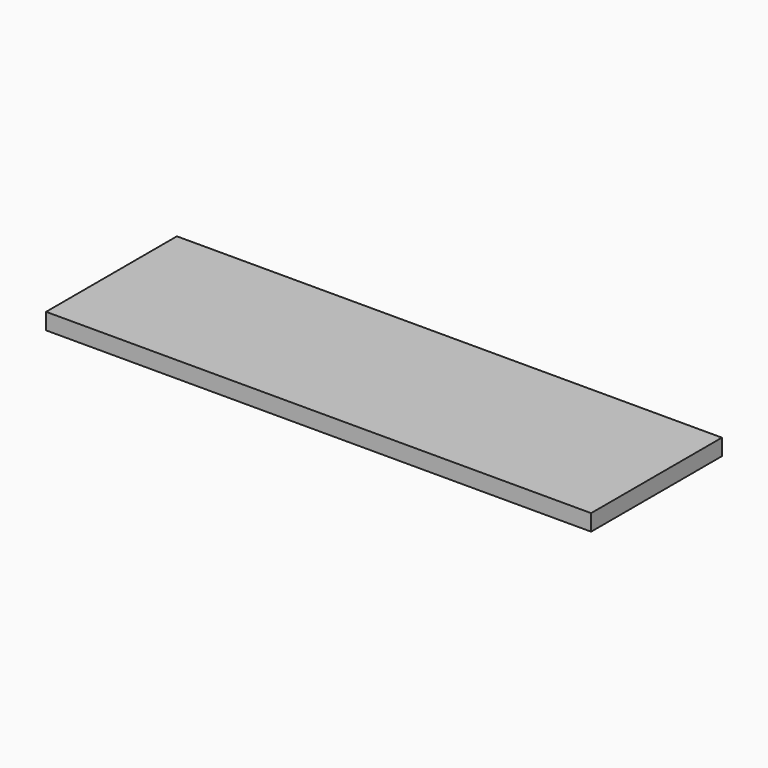
from build123d import *

# Parameters (mm, degrees)
F0_W         = 100
F0_H         = 30
F0_TEXT_SIZE = 22.2058377066
F1_DEPTH     = 2
F2_DEPTH     = 1
F3_W         = 100
F3_H         = 30
F4_DEPTH     = 1


# Not quite as in the source:
# - Text() gives the source's letters only with a copy of the font that has no kerning and outlines rounded to 1/6400 em; it was checked with that copy


with BuildPart() as f1:
    # F0 (on Top) → F1 (new body)
    with BuildSketch(Plane.XY):
        with Locations((-2.6432406157, 9.3667145638)):
            Rectangle(F0_W, F0_H)
        with BuildLine():
            add(Edge.make_bspline(
                [(-36.3527431529, 17.219600889), (-30.4126815664, 17.219600889), (-30.4126815664, 12.6014805785)],
                knots=[0, 0, 0, 1, 1, 1], degree=2))
            add(Edge.make_bspline(
                [(-30.4126815664, 12.6014805785), (-30.4126815664, 10.1935350521), (-32.0555665905, 8.8976162422)],
                knots=[0, 0, 0, 1, 1, 1], degree=2))
            add(Edge.make_bspline(
                [(-32.0555665905, 8.8976162422), (-33.6984516146, 7.6016974323), (-36.7552239613, 7.6016974323)],
                knots=[0, 0, 0, 1, 1, 1], degree=2))
            Line((-36.7552239613, 7.6016974323), (-38.6219021936, 7.6016974323))
            Line((-38.6219021936, 7.6016974323), (-38.6219021936, 1.3667145638))
            Line((-38.6219021936, 1.3667145638), (-40.4642927908, 1.3667145638))
            Line((-40.4642927908, 1.3667145638), (-40.4642927908, 17.219600889))
            Line((-40.4642927908, 17.219600889), (-36.3527431529, 17.219600889))
        make_face(mode=Mode.SUBTRACT)
        with BuildLine():
            add(Edge.make_bspline(
                [(-23.9938066044, 12.8391524352), (-23.0604674883, 13.4688961139), (-21.9432362786, 13.4688961139)],
                knots=[0, 0, 0, 1, 1, 1], degree=2))
            add(Edge.make_bspline(
                [(-21.9432362786, 13.4688961139), (-21.1521533104, 13.4688961139), (-20.5241444627, 13.3370489525)],
                knots=[0, 0, 0, 1, 1, 1], degree=2))
            Line((-20.5241444627, 13.3370489525), (-20.7739601369, 11.6681414623))
            add(Edge.make_bspline(
                [(-20.7739601369, 11.6681414623), (-21.5095285109, 11.831215583), (-22.07508344, 11.831215583)],
                knots=[0, 0, 0, 1, 1, 1], degree=2))
            add(Edge.make_bspline(
                [(-22.07508344, 11.831215583), (-23.518462891, 11.831215583), (-24.5420132227, 10.6602046102)],
                knots=[0, 0, 0, 1, 1, 1], degree=2))
            add(Edge.make_bspline(
                [(-24.5420132227, 10.6602046102), (-25.5655635545, 9.4891936374), (-25.5655635545, 7.7439535801)],
                knots=[0, 0, 0, 1, 1, 1], degree=2))
            Line((-25.5655635545, 7.7439535801), (-25.5655635545, 1.3667145638))
            Line((-25.5655635545, 1.3667145638), (-27.366318206, 1.3667145638))
            Line((-27.366318206, 1.3667145638), (-27.366318206, 13.2503073989))
            Line((-27.366318206, 13.2503073989), (-25.8813028094, 13.2503073989))
            Line((-25.8813028094, 13.2503073989), (-25.6731230809, 11.0505416011))
            Line((-25.6731230809, 11.0505416011), (-25.5863815274, 11.0505416011))
            add(Edge.make_bspline(
                [(-25.5863815274, 11.0505416011), (-24.9271457205, 12.2094087564), (-23.9938066044, 12.8391524352)],
                knots=[0, 0, 0, 1, 1, 1], degree=2))
        make_face(mode=Mode.SUBTRACT)
        with BuildLine():
            add(Edge.make_bspline(
                [(-9.5131716562, 11.8086627791), (-8.0437697392, 10.1484294443), (-8.0437697392, 7.3206547989)],
                knots=[0, 0, 0, 1, 1, 1], degree=2))
            add(Edge.make_bspline(
                [(-8.0437697392, 7.3206547989), (-8.0437697392, 4.4130779242), (-9.5062323319, 2.7806018865)],
                knots=[0, 0, 0, 1, 1, 1], degree=2))
            add(Edge.make_bspline(
                [(-9.5062323319, 2.7806018865), (-10.9686949246, 1.1481258489), (-13.550123558, 1.1481258489)],
                knots=[0, 0, 0, 1, 1, 1], degree=2))
            add(Edge.make_bspline(
                [(-13.550123558, 1.1481258489), (-15.1461681432, 1.1481258489), (-16.3813678656, 1.8975728715)],
                knots=[0, 0, 0, 1, 1, 1], degree=2))
            add(Edge.make_bspline(
                [(-16.3813678656, 1.8975728715), (-17.616567588, 2.6470198941), (-18.2896820435, 4.0452937371)],
                knots=[0, 0, 0, 1, 1, 1], degree=2))
            add(Edge.make_bspline(
                [(-18.2896820435, 4.0452937371), (-18.962796499, 5.4435675802), (-18.962796499, 7.3206547989)],
                knots=[0, 0, 0, 1, 1, 1], degree=2))
            add(Edge.make_bspline(
                [(-18.962796499, 7.3206547989), (-18.962796499, 10.2247620114), (-17.5090080616, 11.8468290626)],
                knots=[0, 0, 0, 1, 1, 1], degree=2))
            add(Edge.make_bspline(
                [(-17.5090080616, 11.8468290626), (-16.0552196243, 13.4688961139), (-13.4737909909, 13.4688961139)],
                knots=[0, 0, 0, 1, 1, 1], degree=2))
            add(Edge.make_bspline(
                [(-13.4737909909, 13.4688961139), (-10.9825735732, 13.4688961139), (-9.5131716562, 11.8086627791)],
                knots=[0, 0, 0, 1, 1, 1], degree=2))
        make_face(mode=Mode.SUBTRACT)
        with BuildLine():
            add(Edge.make_bspline(
                [(-2.4472047047, 3.2108399921), (-1.9371643699, 2.6366109076), (-1.0489308616, 2.6366109076)],
                knots=[0, 0, 0, 1, 1, 1], degree=2))
            add(Edge.make_bspline(
                [(-1.0489308616, 2.6366109076), (-0.5701174861, 2.6366109076), (-0.126000732, 2.7060041505)],
                knots=[0, 0, 0, 1, 1, 1], degree=2))
            add(Edge.make_bspline(
                [(-0.126000732, 2.7060041505), (0.3181160222, 2.7753973933), (0.5783406828, 2.8517299604)],
                knots=[0, 0, 0, 1, 1, 1], degree=2))
            Line((0.5783406828, 2.8517299604), (0.5783406828, 1.4742740902))
            add(Edge.make_bspline(
                [(0.5783406828, 1.4742740902), (0.2868890629, 1.3354876045), (-0.2821355283, 1.2418067267)],
                knots=[0, 0, 0, 1, 1, 1], degree=2))
            add(Edge.make_bspline(
                [(-0.2821355283, 1.2418067267), (-0.8511601196, 1.1481258489), (-1.3091555223, 1.1481258489)],
                knots=[0, 0, 0, 1, 1, 1], degree=2))
            add(Edge.make_bspline(
                [(-1.3091555223, 1.1481258489), (-4.7545300289, 1.1481258489), (-4.7545300289, 4.7808621112)],
                knots=[0, 0, 0, 1, 1, 1], degree=2))
            Line((-4.7545300289, 4.7808621112), (-4.7545300289, 11.8520335559))
            Line((-4.7545300289, 11.8520335559), (-6.4581341405, 11.8520335559))
            Line((-6.4581341405, 11.8520335559), (-6.4581341405, 12.7194490913))
            Line((-6.4581341405, 12.7194490913), (-4.7545300289, 13.4688961139))
            Line((-4.7545300289, 13.4688961139), (-3.998143682, 16.0052191394))
            Line((-3.998143682, 16.0052191394), (-2.9572450395, 16.0052191394))
            Line((-2.9572450395, 16.0052191394), (-2.9572450395, 13.2503073989))
            Line((-2.9572450395, 13.2503073989), (0.4915991293, 13.2503073989))
            Line((0.4915991293, 13.2503073989), (0.4915991293, 11.8520335559))
            Line((0.4915991293, 11.8520335559), (-2.9572450395, 11.8520335559))
            Line((-2.9572450395, 11.8520335559), (-2.9572450395, 4.8571946783))
            add(Edge.make_bspline(
                [(-2.9572450395, 4.8571946783), (-2.9572450395, 3.7850690765), (-2.4472047047, 3.2108399921)],
                knots=[0, 0, 0, 1, 1, 1], degree=2))
        make_face(mode=Mode.SUBTRACT)
        with BuildLine():
            add(Edge.make_bspline(
                [(10.0262306945, 1.3285482802), (9.1761634698, 1.1481258489), (7.9721907066, 1.1481258489)],
                knots=[0, 0, 0, 1, 1, 1], degree=2))
            add(Edge.make_bspline(
                [(7.9721907066, 1.1481258489), (5.3387171411, 1.1481258489), (3.8138006299, 2.7545794205)],
                knots=[0, 0, 0, 1, 1, 1], degree=2))
            add(Edge.make_bspline(
                [(3.8138006299, 2.7545794205), (2.2888841186, 4.361032992), (2.2888841186, 7.2096256103)],
                knots=[0, 0, 0, 1, 1, 1], degree=2))
            add(Edge.make_bspline(
                [(2.2888841186, 7.2096256103), (2.2888841186, 10.0859755258), (3.7045062724, 11.7774358198)],
                knots=[0, 0, 0, 1, 1, 1], degree=2))
            add(Edge.make_bspline(
                [(3.7045062724, 11.7774358198), (5.1201284262, 13.4688961139), (7.5072559797, 13.4688961139)],
                knots=[0, 0, 0, 1, 1, 1], degree=2))
            add(Edge.make_bspline(
                [(7.5072559797, 13.4688961139), (9.7382487367, 13.4688961139), (11.0393720399, 11.9994941969)],
                knots=[0, 0, 0, 1, 1, 1], degree=2))
            add(Edge.make_bspline(
                [(11.0393720399, 11.9994941969), (12.340495343, 10.5300922799), (12.340495343, 8.1221467536)],
                knots=[0, 0, 0, 1, 1, 1], degree=2))
            Line((12.340495343, 8.1221467536), (12.340495343, 6.9840975711))
            Line((12.340495343, 6.9840975711), (4.1555623508, 6.9840975711))
            add(Edge.make_bspline(
                [(4.1555623508, 6.9840975711), (4.2110769451, 4.8918912997), (5.213809304, 3.8076218804)],
                knots=[0, 0, 0, 1, 1, 1], degree=2))
            add(Edge.make_bspline(
                [(5.213809304, 3.8076218804), (6.216541663, 2.7233524612), (8.0381142873, 2.7233524612)],
                knots=[0, 0, 0, 1, 1, 1], degree=2))
            add(Edge.make_bspline(
                [(8.0381142873, 2.7233524612), (9.9568374517, 2.7233524612), (11.8304550082, 3.5248444159)],
                knots=[0, 0, 0, 1, 1, 1], degree=2))
            Line((11.8304550082, 3.5248444159), (11.8304550082, 1.9183908443))
            add(Edge.make_bspline(
                [(11.8304550082, 1.9183908443), (10.8762979192, 1.5089707116), (10.0262306945, 1.3285482802)],
                knots=[0, 0, 0, 1, 1, 1], degree=2))
        make_face(mode=Mode.SUBTRACT)
        with BuildLine():
            add(Edge.make_bspline(
                [(23.1623715628, 1.7691953722), (21.9722774482, 1.1481258489), (20.1611138103, 1.1481258489)],
                knots=[0, 0, 0, 1, 1, 1], degree=2))
            add(Edge.make_bspline(
                [(20.1611138103, 1.1481258489), (17.5796851769, 1.1481258489), (16.1640630231, 2.7372311097)],
                knots=[0, 0, 0, 1, 1, 1], degree=2))
            add(Edge.make_bspline(
                [(16.1640630231, 2.7372311097), (14.7484408693, 4.3263363706), (14.7484408693, 7.2339132453)],
                knots=[0, 0, 0, 1, 1, 1], degree=2))
            add(Edge.make_bspline(
                [(14.7484408693, 7.2339132453), (14.7484408693, 10.214353025), (16.186615827, 11.8416245694)],
                knots=[0, 0, 0, 1, 1, 1], degree=2))
            add(Edge.make_bspline(
                [(16.186615827, 11.8416245694), (17.6247907847, 13.4688961139), (20.2790823231, 13.4688961139)],
                knots=[0, 0, 0, 1, 1, 1], degree=2))
            add(Edge.make_bspline(
                [(20.2790823231, 13.4688961139), (21.1360888721, 13.4688961139), (21.9930954211, 13.2832691893)],
                knots=[0, 0, 0, 1, 1, 1], degree=2))
            add(Edge.make_bspline(
                [(21.9930954211, 13.2832691893), (22.85010197, 13.0976422647), (23.3358546699, 12.8478265905)],
                knots=[0, 0, 0, 1, 1, 1], degree=2))
            Line((23.3358546699, 12.8478265905), (22.7841783893, 11.3211752482))
            add(Edge.make_bspline(
                [(22.7841783893, 11.3211752482), (22.187396501, 11.560581936), (21.4830550862, 11.7167167323)],
                knots=[0, 0, 0, 1, 1, 1], degree=2))
            add(Edge.make_bspline(
                [(21.4830550862, 11.7167167323), (20.7787136715, 11.8728515287), (20.2374463774, 11.8728515287)],
                knots=[0, 0, 0, 1, 1, 1], degree=2))
            add(Edge.make_bspline(
                [(20.2374463774, 11.8728515287), (16.6151191015, 11.8728515287), (16.6151191015, 7.2547312182)],
                knots=[0, 0, 0, 1, 1, 1], degree=2))
            add(Edge.make_bspline(
                [(16.6151191015, 7.2547312182), (16.6151191015, 5.0653744068), (17.4981481165, 3.894363434)],
                knots=[0, 0, 0, 1, 1, 1], degree=2))
            add(Edge.make_bspline(
                [(17.4981481165, 3.894363434), (18.3811771316, 2.7233524612), (20.1160082024, 2.7233524612)],
                knots=[0, 0, 0, 1, 1, 1], degree=2))
            add(Edge.make_bspline(
                [(20.1160082024, 2.7233524612), (21.601023599, 2.7233524612), (23.1623715628, 3.3617702952)],
                knots=[0, 0, 0, 1, 1, 1], degree=2))
            Line((23.1623715628, 3.3617702952), (23.1623715628, 1.7691953722))
        make_face(mode=Mode.SUBTRACT)
        with BuildLine():
            Line((35.9168495955, 1.3667145638), (34.116094944, 1.3667145638))
            Line((34.116094944, 1.3667145638), (34.116094944, 9.0554858697))
            add(Edge.make_bspline(
                [(34.116094944, 9.0554858697), (34.116094944, 10.5058046449), (33.455124306, 11.2222898771)],
                knots=[0, 0, 0, 1, 1, 1], degree=2))
            add(Edge.make_bspline(
                [(33.455124306, 11.2222898771), (32.794153668, 11.9387751094), (31.3820011764, 11.9387751094)],
                knots=[0, 0, 0, 1, 1, 1], degree=2))
            add(Edge.make_bspline(
                [(31.3820011764, 11.9387751094), (29.5083836199, 11.9387751094), (28.6461725777, 10.9186944398)],
                knots=[0, 0, 0, 1, 1, 1], degree=2))
            add(Edge.make_bspline(
                [(28.6461725777, 10.9186944398), (27.7839615355, 9.8986137701), (27.7839615355, 7.5808794595)],
                knots=[0, 0, 0, 1, 1, 1], degree=2))
            Line((27.7839615355, 7.5808794595), (27.7839615355, 1.3667145638))
            Line((27.7839615355, 1.3667145638), (25.9832068839, 1.3667145638))
            Line((25.9832068839, 1.3667145638), (25.9832068839, 18.2396815586))
            Line((25.9832068839, 18.2396815586), (27.7839615355, 18.2396815586))
            Line((27.7839615355, 18.2396815586), (27.7839615355, 13.1323388861))
            add(Edge.make_bspline(
                [(27.7839615355, 13.1323388861), (27.7839615355, 12.2094087564), (27.6972199819, 11.6022178817)],
                knots=[0, 0, 0, 1, 1, 1], degree=2))
            Line((27.6972199819, 11.6022178817), (27.8047795083, 11.6022178817))
            add(Edge.make_bspline(
                [(27.8047795083, 11.6022178817), (28.335637816, 12.4592244306), (29.3175522021, 12.9519164548)],
                knots=[0, 0, 0, 1, 1, 1], degree=2))
            add(Edge.make_bspline(
                [(29.3175522021, 12.9519164548), (30.2994665882, 13.4446084789), (31.5554842834, 13.4446084789)],
                knots=[0, 0, 0, 1, 1, 1], degree=2))
            add(Edge.make_bspline(
                [(31.5554842834, 13.4446084789), (33.7344321084, 13.4446084789), (34.8256408519, 12.4089143296)],
                knots=[0, 0, 0, 1, 1, 1], degree=2))
            add(Edge.make_bspline(
                [(34.8256408519, 12.4089143296), (35.9168495955, 11.3732201803), (35.9168495955, 9.1179397882)],
                knots=[0, 0, 0, 1, 1, 1], degree=2))
            Line((35.9168495955, 9.1179397882), (35.9168495955, 1.3667145638))
        make_face(mode=Mode.SUBTRACT)
        with BuildLine():
            add(Edge.make_bspline(
                [(-16.195740941, 10.778173123), (-17.0961182668, 9.6175711366), (-17.0961182668, 7.3206547989)],
                knots=[0, 0, 0, 1, 1, 1], degree=2))
            add(Edge.make_bspline(
                [(-17.0961182668, 7.3206547989), (-17.0961182668, 5.0410867718), (-16.1853319546, 3.8492578261)],
                knots=[0, 0, 0, 1, 1, 1], degree=2))
            add(Edge.make_bspline(
                [(-16.1853319546, 3.8492578261), (-15.2745456424, 2.6574288805), (-13.5084876123, 2.6574288805)],
                knots=[0, 0, 0, 1, 1, 1], degree=2))
            add(Edge.make_bspline(
                [(-13.5084876123, 2.6574288805), (-11.7389599201, 2.6574288805), (-10.8229691147, 3.8440533329)],
                knots=[0, 0, 0, 1, 1, 1], degree=2))
            add(Edge.make_bspline(
                [(-10.8229691147, 3.8440533329), (-9.9069783093, 5.0306777854), (-9.9069783093, 7.3206547989)],
                knots=[0, 0, 0, 1, 1, 1], degree=2))
            add(Edge.make_bspline(
                [(-9.9069783093, 7.3206547989), (-9.9069783093, 9.5863441774), (-10.8229691147, 10.7625596434)],
                knots=[0, 0, 0, 1, 1, 1], degree=2))
            add(Edge.make_bspline(
                [(-10.8229691147, 10.7625596434), (-11.7389599201, 11.9387751094), (-13.5293055851, 11.9387751094)],
                knots=[0, 0, 0, 1, 1, 1], degree=2))
            add(Edge.make_bspline(
                [(-13.5293055851, 11.9387751094), (-15.2953636152, 11.9387751094), (-16.195740941, 10.778173123)],
                knots=[0, 0, 0, 1, 1, 1], degree=2))
        make_face()
        with BuildLine():
            Line((-38.6219021936, 15.6235563038), (-38.6219021936, 9.1838633689))
            Line((-38.6219021936, 9.1838633689), (-36.9599340277, 9.1838633689))
            add(Edge.make_bspline(
                [(-36.9599340277, 9.1838633689), (-34.5103525557, 9.1838633689), (-33.41567415, 9.9749463372)],
                knots=[0, 0, 0, 1, 1, 1], degree=2))
            add(Edge.make_bspline(
                [(-33.41567415, 9.9749463372), (-32.3209957443, 10.7660293055), (-32.3209957443, 12.5147390249)],
                knots=[0, 0, 0, 1, 1, 1], degree=2))
            add(Edge.make_bspline(
                [(-32.3209957443, 12.5147390249), (-32.3209957443, 14.0864959751), (-33.3514854004, 14.8550261395)],
                knots=[0, 0, 0, 1, 1, 1], degree=2))
            add(Edge.make_bspline(
                [(-33.3514854004, 14.8550261395), (-34.3819750565, 15.6235563038), (-36.5609228814, 15.6235563038)],
                knots=[0, 0, 0, 1, 1, 1], degree=2))
            Line((-36.5609228814, 15.6235563038), (-38.6219021936, 15.6235563038))
        make_face()
        with Locations((-42.6432406157, 1.3667145638)):
            Text('Protech', F0_TEXT_SIZE, font='Open Sans', text_align=(TextAlign.LEFT, TextAlign.BOTTOM))
        with BuildLine():
            add(Edge.make_bspline(
                [(9.6532420143, 11.0540112633), (8.8951208363, 11.9595930822), (7.4829683447, 11.9595930822)],
                knots=[0, 0, 0, 1, 1, 1], degree=2))
            add(Edge.make_bspline(
                [(7.4829683447, 11.9595930822), (6.0534675423, 11.9595930822), (5.2016654865, 11.0279887972)],
                knots=[0, 0, 0, 1, 1, 1], degree=2))
            add(Edge.make_bspline(
                [(5.2016654865, 11.0279887972), (4.3498634308, 10.0963845122), (4.1971982965, 8.4482949949)],
                knots=[0, 0, 0, 1, 1, 1], degree=2))
            Line((4.1971982965, 8.4482949949), (10.4113631922, 8.4482949949))
            add(Edge.make_bspline(
                [(10.4113631922, 8.4482949949), (10.4113631922, 10.1484294443), (9.6532420143, 11.0540112633)],
                knots=[0, 0, 0, 1, 1, 1], degree=2))
        make_face()
    extrude(amount=-F1_DEPTH)

    # F0 (on Top) → F2 (cut)
    with BuildSketch(Plane.XY):
        with Locations((-42.6432406157, 1.3667145638)):
            Text('Protech', F0_TEXT_SIZE, font='Open Sans', text_align=(TextAlign.LEFT, TextAlign.BOTTOM))
    extrude(amount=-F2_DEPTH, mode=Mode.SUBTRACT)

    # F3 (on face) → F4 (join)
    with BuildSketch(Plane.XY):
        with Locations((-2.6432406157, 9.3667145638)):
            Rectangle(F3_W, F3_H)
    extrude(amount=F4_DEPTH)


solid = f1.part
